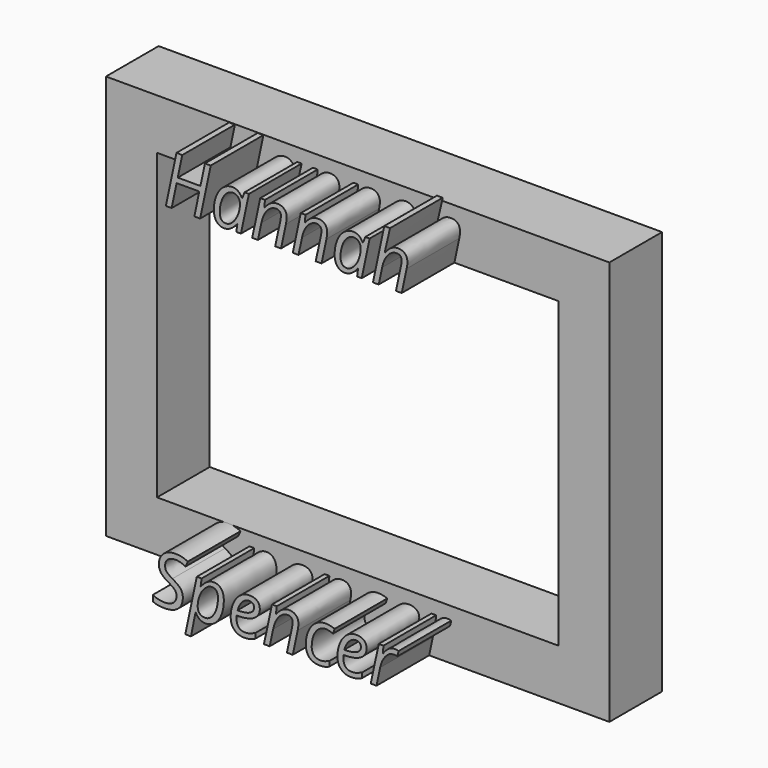
from build123d import *

# Parameters (mm, degrees)
F0_W         = 194.1799372435
F0_H         = 156.0077667236
F0_W_2       = 154.7629833221
F0_H_2       = 117.0058250427
F1_DEPTH     = 25.4
F2_TEXT_SIZE = 27.0846817229
F3_DEPTH     = 25.4
F4_TEXT_SIZE = 27.0846817229
F5_DEPTH     = 25.4


# Not quite as in the source:
# - Text() gives the source's letters only with a copy of the font that has no kerning and outlines rounded to 1/6400 em; it was checked with that copy


with BuildPart() as f1:
    # F0 (on Front) → F1 (new body)
    with BuildSketch(Plane.XZ):
        with Locations((0, 18.878608942)):
            Rectangle(F0_W, F0_H)
        with Locations((0, 18.878608942)):
            Rectangle(F0_W_2, F0_H_2, mode=Mode.SUBTRACT)
    extrude(amount=F1_DEPTH)

    # F2 (on face) → F3 (join)
    with BuildSketch(Plane.XZ.offset(25.4)):
        with Locations((-54.8036430135, 77.3815214634)):
            Text('Hannah', F2_TEXT_SIZE, font='Open Sans', font_style=FontStyle.ITALIC, text_align=(TextAlign.LEFT, TextAlign.BOTTOM))
    extrude(amount=F3_DEPTH)

    # F4 (on face) → F5 (join)
    with BuildSketch(Plane.XZ.offset(25.4)):
        with Locations((-59.1903586044, -59.1252744198)):
            Text('Spencer', F4_TEXT_SIZE, font='Open Sans', font_style=FontStyle.ITALIC, text_align=(TextAlign.LEFT, TextAlign.BOTTOM))
    extrude(amount=F5_DEPTH)


solid = f1.part
